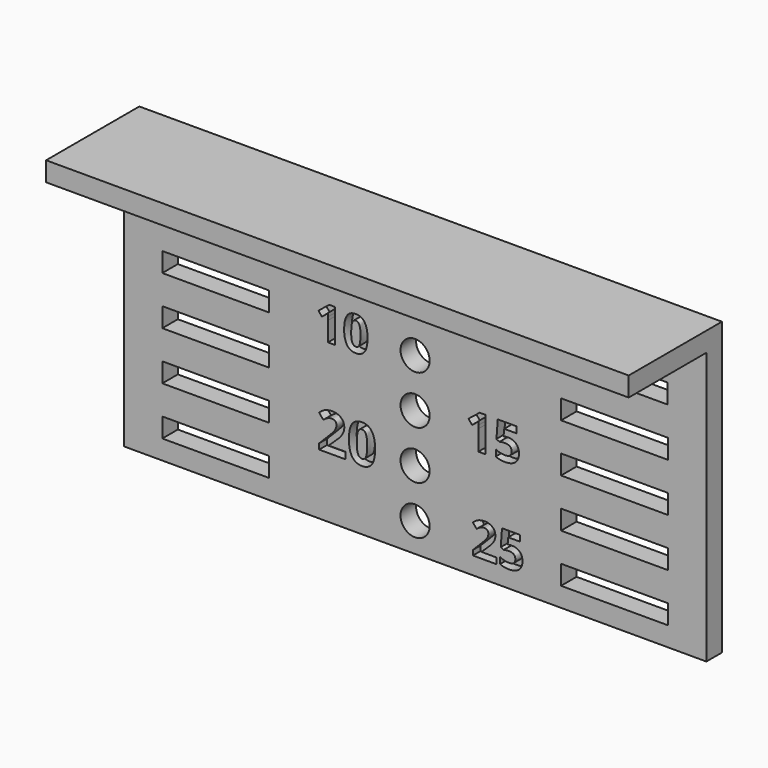
from build123d import *

# Parameters (mm, degrees)
F0_W          = 60
F0_H          = 30
F1_DEPTH      = 2
F2_W          = 60
F2_H          = 2
F3_DEPTH      = 10
F4_W          = 11
F4_H          = 1
F5_DEPTH      = 3
F6_W          = 11
F6_H          = 1
F7_DEPTH      = 25
F8_W          = 11
F8_H          = 1
F9_DEPTH      = 25
F10_W         = 11
F10_H         = 1
F11_DEPTH     = 25
F12_W         = 11
F12_H         = 1
F13_DEPTH     = 25
F14_TEXT_SIZE = 5.6034012232
F15_DEPTH     = 1
F16_TEXT_SIZE = 4.830517638
F17_DEPTH     = 1
F18_TEXT_SIZE = 5.0089331732
F19_DEPTH     = 1
F20_TEXT_SIZE = 5.4101789525
F21_DEPTH     = 1
F22_TEXT_SIZE = 4.8305166678
F23_DEPTH     = 1


# Not quite as in the source:
# - Text() gives the source's letters only with a copy of the font that has no kerning and outlines rounded to 1/6400 em; it was checked with that copy


with BuildPart() as f1:
    # F0 (on Front) → F1 (new body)
    with BuildSketch(Plane.XZ):
        Rectangle(F0_W, F0_H)
    extrude(amount=F1_DEPTH)

    # F2 (on face) → F3 (join)
    with BuildSketch(Plane.XZ.offset(2)):
        with Locations((0, 14)):
            Rectangle(F2_W, F2_H)
    extrude(amount=F3_DEPTH)

    # F4 (on face) → F5 (cut)
    with BuildSketch(Plane.XZ.offset(2)):
        with Locations((20.5, 8.5)):
            Rectangle(F4_W, F4_H)
        with Locations((20.5, 7.5)):
            Rectangle(F4_W, F4_H)
        with BuildLine():
            Line((1.5, 8), (-1.5, 8))
            ThreePointArc((-1.5, 8), (0, 6.5), (1.5, 8))
        make_face()
        with BuildLine():
            ThreePointArc((1.5, 8), (0, 9.5), (-1.5, 8))
            Line((-1.5, 8), (1.5, 8))
        make_face()
        with Locations((-20.5, 8.5)):
            Rectangle(F4_W, F4_H)
        with Locations((-20.5, 7.5)):
            Rectangle(F4_W, F4_H)
    extrude(amount=-F5_DEPTH, mode=Mode.SUBTRACT)

    # F6 (on face) → F7 (cut)
    with BuildSketch(Plane.XZ.offset(2)):
        with Locations((-20.5315700102, 3.5)):
            Rectangle(F6_W, F6_H)
        with Locations((20.5315700102, 3.5)):
            Rectangle(F6_W, F6_H)
        with Locations((20.5315700102, 2.5)):
            Rectangle(F6_W, F6_H)
        with BuildLine():
            ThreePointArc((1.5, 3), (0, 4.5), (-1.5, 3))
            Line((-1.5, 3), (1.5, 3))
        make_face()
        with BuildLine():
            Line((1.5, 3), (-1.5, 3))
            ThreePointArc((-1.5, 3), (0, 1.5), (1.5, 3))
        make_face()
        with Locations((-20.5315700102, 2.5)):
            Rectangle(F6_W, F6_H)
    extrude(amount=-F7_DEPTH, mode=Mode.SUBTRACT)

    # F8 (on face) → F9 (cut)
    with BuildSketch(Plane.XZ.offset(2)):
        with Locations((-20.5315700102, -1.5)):
            Rectangle(F8_W, F8_H)
        with Locations((20.5315700102, -1.5)):
            Rectangle(F8_W, F8_H)
        with Locations((20.5315700102, -2.5)):
            Rectangle(F8_W, F8_H)
        with BuildLine():
            ThreePointArc((1.5, -2), (0, -0.5), (-1.5, -2))
            Line((-1.5, -2), (1.5, -2))
        make_face()
        with BuildLine():
            Line((1.5, -2), (-1.5, -2))
            ThreePointArc((-1.5, -2), (0, -3.5), (1.5, -2))
        make_face()
        with Locations((-20.5315700102, -2.5)):
            Rectangle(F8_W, F8_H)
    extrude(amount=-F9_DEPTH, mode=Mode.SUBTRACT)

    # F10 (on face) → F11 (cut)
    with BuildSketch(Plane.XZ.offset(2)):
        with Locations((-20.5315700102, -6.5)):
            Rectangle(F10_W, F10_H)
        with Locations((20.5315700102, -6.5)):
            Rectangle(F10_W, F10_H)
        with Locations((20.5315700102, -7.5)):
            Rectangle(F10_W, F10_H)
        with BuildLine():
            ThreePointArc((1.5, -7), (0, -5.5), (-1.5, -7))
            Line((-1.5, -7), (1.5, -7))
        make_face()
        with BuildLine():
            Line((1.5, -7), (-1.5, -7))
            ThreePointArc((-1.5, -7), (0, -8.5), (1.5, -7))
        make_face()
        with Locations((-20.5315700102, -7.5)):
            Rectangle(F10_W, F10_H)
    extrude(amount=-F11_DEPTH, mode=Mode.SUBTRACT)

    # F12 (on face) → F13 (cut)
    with BuildSketch(Plane.XZ.offset(2)):
        with Locations((-20.5315700102, -11.5)):
            Rectangle(F12_W, F12_H)
        with Locations((20.5315700102, -11.5)):
            Rectangle(F12_W, F12_H)
        with Locations((20.5315700102, -12.5)):
            Rectangle(F12_W, F12_H)
        with BuildLine():
            ThreePointArc((1.5, -12), (0, -10.5), (-1.5, -12))
            Line((-1.5, -12), (1.5, -12))
        make_face()
        with BuildLine():
            Line((1.5, -12), (-1.5, -12))
            ThreePointArc((-1.5, -12), (0, -13.5), (1.5, -12))
        make_face()
        with Locations((-20.5315700102, -12.5)):
            Rectangle(F12_W, F12_H)
    extrude(amount=-F13_DEPTH, mode=Mode.SUBTRACT)

    # F14 (on face) → F15 (cut)
    with BuildSketch(Plane.XZ.offset(2)):
        with Locations((4.2320485227, 6.4101289026)):
            Text('5', F14_TEXT_SIZE, font='Open Sans', font_style=FontStyle.BOLD, text_align=(TextAlign.LEFT, TextAlign.BOTTOM))
    extrude(amount=-F15_DEPTH, mode=Mode.SUBTRACT)

    # F16 (on face) → F17 (cut)
    with BuildSketch(Plane.XZ.offset(2)):
        with Locations((-10.2363163605, 1.2627297547)):
            Text('10', F16_TEXT_SIZE, font='Open Sans', font_style=FontStyle.BOLD, text_align=(TextAlign.LEFT, TextAlign.BOTTOM))
    extrude(amount=-F17_DEPTH, mode=Mode.SUBTRACT)

    # F18 (on face) → F19 (cut)
    with BuildSketch(Plane.XZ.offset(2)):
        with Locations((5.2058813162, -3.6064318847)):
            Text('15', F18_TEXT_SIZE, font='Open Sans', font_style=FontStyle.BOLD, text_align=(TextAlign.LEFT, TextAlign.BOTTOM))
    extrude(amount=-F19_DEPTH, mode=Mode.SUBTRACT)

    # F20 (on face) → F21 (cut)
    with BuildSketch(Plane.XZ.offset(2)):
        with Locations((-10.0971981883, -8.7538310327)):
            Text('20', F20_TEXT_SIZE, font='Open Sans', font_style=FontStyle.BOLD, text_align=(TextAlign.LEFT, TextAlign.BOTTOM))
    extrude(amount=-F21_DEPTH, mode=Mode.SUBTRACT)

    # F22 (on face) → F23 (cut)
    with BuildSketch(Plane.XZ.offset(2)):
        with Locations((5.7623567991, -13.2056353614)):
            Text('25', F22_TEXT_SIZE, font='Open Sans', font_style=FontStyle.BOLD, text_align=(TextAlign.LEFT, TextAlign.BOTTOM))
    extrude(amount=-F23_DEPTH, mode=Mode.SUBTRACT)


solid = f1.part
